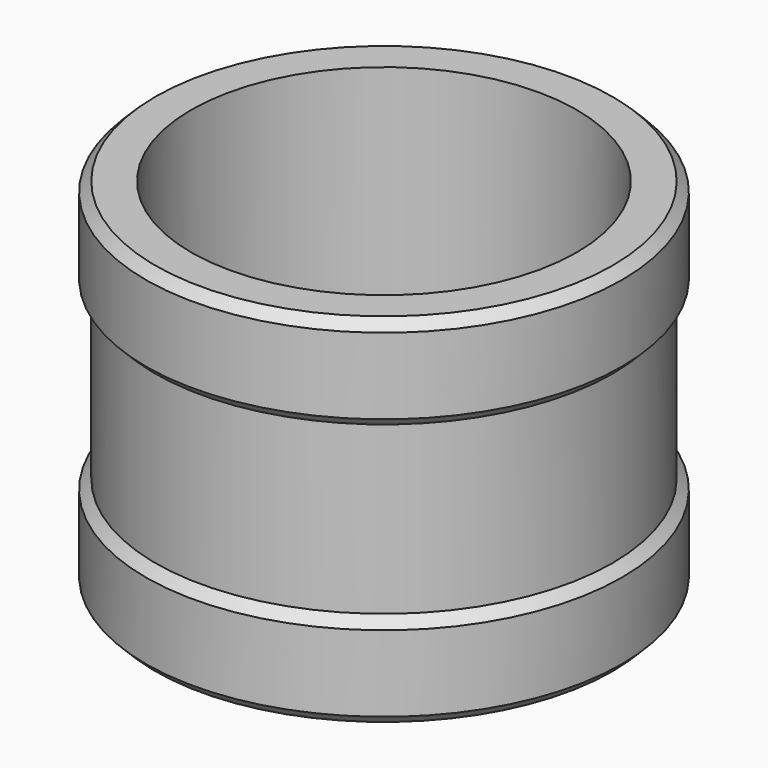
from build123d import *

# Parameters (mm, degrees)
F0_R     = 6.096
F0_R_2   = 5.1435
F1_DEPTH = 9.525
F2_R     = 6.35
F2_R_2   = 5.1435
F3_DEPTH = 2.54
F4_R     = 6.35
F4_R_2   = 5.1435
F5_DEPTH = 2.54
F6_SIZE  = 0.25399


# Not quite as in the source:
# - a fillet or chamfer is up to 0.001 mm smaller than in the source, because OpenCascade refuses the exact size


with BuildPart() as f1:
    # F0 (on Top) → F1 (new body)
    with BuildSketch(Plane.XY):
        Circle(F0_R)
        Circle(F0_R_2, mode=Mode.SUBTRACT)
    extrude(amount=F1_DEPTH)

    # F2 (on face) → F3 (join)
    with BuildSketch(Plane.XY.offset(9.525)):
        Circle(F2_R)
        Circle(F2_R_2, mode=Mode.SUBTRACT)
    extrude(amount=-F3_DEPTH)

    # F4 (on face) → F5 (join)
    with BuildSketch(Plane(origin=(0, 0, 0), x_dir=(1, 0, 0), z_dir=(0, 0, -1))):
        Circle(F4_R)
        Circle(F4_R_2, mode=Mode.SUBTRACT)
    extrude(amount=-F5_DEPTH)

    # F6 (size 0.254 in the source; OpenCascade refuses exactly that, so slightly less here)
    f6_edges = [f1.edges().sort_by_distance(p)[0] for p in [
        (-6.35, 0, 6.985),
        (-6.35, 0, 9.525),
        (-6.35, 0, 2.54),
        (-6.35, 0, 0),
    ]]
    chamfer(f6_edges, length=F6_SIZE)


solid = f1.part
